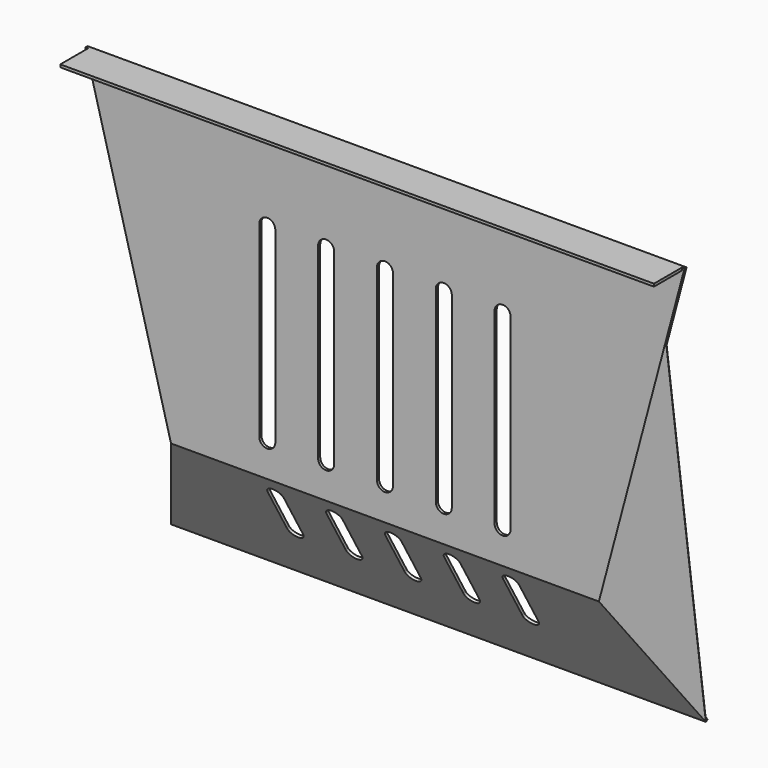
from build123d import *

# Parameters (mm, degrees)
F1_DEPTH = 0.5
F2_W     = 111
F2_H     = 0.5
F3_DEPTH = 6.5
F6_DEPTH = 0.5
F9_DEPTH = 0.5


# Not quite as in the source:
# - a feature of the source that left no trace in its solid (it failed there, or was rolled back) is left out


with BuildPart() as f1:
    # F0 (on Front) → F1 (new body)
    with BuildSketch(Plane.XZ):
        Polygon((-40, 0), (40, 0), (56, 60), (-56, 60), align=None)
        with BuildLine():
            Line((-20.5, 41.5), (-20.5, 6.5))
            ThreePointArc((-20.5, 6.5), (-22, 5), (-23.5, 6.5))
            Line((-23.5, 6.5), (-23.5, 41.5))
            ThreePointArc((-23.5, 41.5), (-22, 43), (-20.5, 41.5))
        make_face(mode=Mode.SUBTRACT)
        with BuildLine():
            Line((-9.5, 41.5), (-9.5, 6.5))
            ThreePointArc((-9.5, 6.5), (-11, 5), (-12.5, 6.5))
            Line((-12.5, 6.5), (-12.5, 41.5))
            ThreePointArc((-12.5, 41.5), (-11, 43), (-9.5, 41.5))
        make_face(mode=Mode.SUBTRACT)
        with BuildLine():
            Line((1.5, 41.5), (1.5, 6.5))
            ThreePointArc((1.5, 6.5), (0, 5), (-1.5, 6.5))
            Line((-1.5, 6.5), (-1.5, 41.5))
            ThreePointArc((-1.5, 41.5), (0, 43), (1.5, 41.5))
        make_face(mode=Mode.SUBTRACT)
        with BuildLine():
            Line((12.5, 41.5), (12.5, 6.5))
            ThreePointArc((12.5, 6.5), (11, 5), (9.5, 6.5))
            Line((9.5, 6.5), (9.5, 41.5))
            ThreePointArc((9.5, 41.5), (11, 43), (12.5, 41.5))
        make_face(mode=Mode.SUBTRACT)
        with BuildLine():
            Line((20.5, 6.5), (20.5, 41.5))
            ThreePointArc((20.5, 41.5), (22, 43), (23.5, 41.5))
            Line((23.5, 41.5), (23.5, 6.5))
            ThreePointArc((23.5, 6.5), (22, 5), (20.5, 6.5))
        make_face(mode=Mode.SUBTRACT)
    extrude(amount=F1_DEPTH)

    # F2 (on face) → F3 (join)
    with BuildSketch(Plane.XZ.offset(0.5)):
        with Locations((0, 59.75)):
            Rectangle(F2_W, F2_H)
    extrude(amount=F3_DEPTH)

    # F5 (on face) → F6 (join)
    with BuildSketch(Plane(origin=(0, -0.375, -0.2165063509), x_dir=(1, 0, 0), z_dir=(0, -0.8660254038, -0.5))):
        Polygon((50, -24.75), (40, 0.25), (-40, 0.25), (-50, -24.75), align=None)
        with BuildLine():
            Line((-23.5, -12.75), (-23.5, -3.75))
            ThreePointArc((-23.5, -3.75), (-22, -2.25), (-20.5, -3.75))
            Line((-20.5, -3.75), (-20.5, -12.75))
            ThreePointArc((-20.5, -12.75), (-22, -14.25), (-23.5, -12.75))
        make_face(mode=Mode.SUBTRACT)
        with BuildLine():
            ThreePointArc((-9.5, -12.75), (-11, -14.25), (-12.5, -12.75))
            Line((-12.5, -12.75), (-12.5, -3.75))
            ThreePointArc((-12.5, -3.75), (-11, -2.25), (-9.5, -3.75))
            Line((-9.5, -3.75), (-9.5, -12.75))
        make_face(mode=Mode.SUBTRACT)
        with BuildLine():
            ThreePointArc((1.5, -12.75), (0, -14.25), (-1.5, -12.75))
            Line((-1.5, -12.75), (-1.5, -3.75))
            ThreePointArc((-1.5, -3.75), (0, -2.25), (1.5, -3.75))
            Line((1.5, -3.75), (1.5, -12.75))
        make_face(mode=Mode.SUBTRACT)
        with BuildLine():
            ThreePointArc((12.5, -12.75), (11, -14.25), (9.5, -12.75))
            Line((9.5, -12.75), (9.5, -3.75))
            ThreePointArc((9.5, -3.75), (11, -2.25), (12.5, -3.75))
            Line((12.5, -3.75), (12.5, -12.75))
        make_face(mode=Mode.SUBTRACT)
        with BuildLine():
            ThreePointArc((23.5, -12.75), (22, -14.25), (20.5, -12.75))
            Line((20.5, -12.75), (20.5, -3.75))
            ThreePointArc((20.5, -3.75), (22, -2.25), (23.5, -3.75))
            Line((23.5, -3.75), (23.5, -12.75))
        make_face(mode=Mode.SUBTRACT)
    extrude(amount=-F6_DEPTH)

    # F8 (on 3pt) → F9 (join)
    with BuildSketch(Plane(origin=(15.2549879147, -19.249967435, -4.0679967773), x_dir=(-0.7902831791, -0.5995016599, -0.1266896076), z_dir=(-0.6127417865, 0.7732067375, 0.1633978097))):
        Polygon((-47.1762423682, 46.1033792785), (-43.9652684076, -23.663910783), (-31.3115763324, 0.1033792785), align=None)
    extrude(amount=F9_DEPTH)


solid = f1.part
